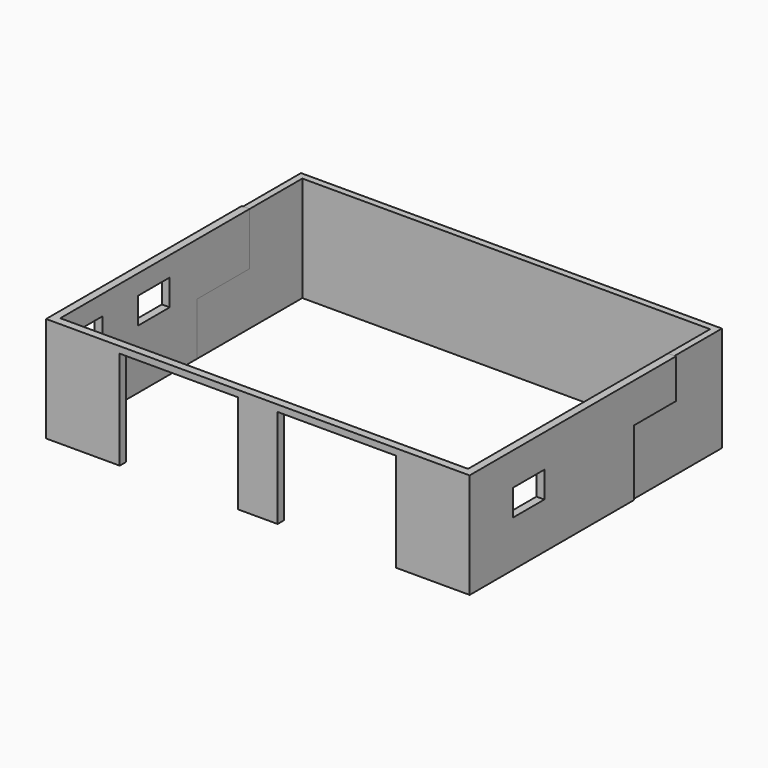
from build123d import *

# Parameters (mm, degrees)
F0_W           = 9753.6
F0_H           = 7315.2
F1_DEPTH       = 304.8
F2_W           = 914.4
F2_H           = 152.4
F3_DEPTH       = 152.4
F5_DEPTH       = 2438.4
F7_DEPTH       = 152.4
F9_DEPTH       = 152.4
F10_W          = 914.4
F10_H          = 609.6
F11_DEPTH      = 152.4
F11_DEPTH_BACK = 30.48
F13_DEPTH      = 152.4
F13_DEPTH_BACK = 30.48
F14_W          = 914.4
F14_H          = 609.6
F15_DEPTH      = 182.88
F16_W          = 9753.6
F16_H          = 7315.2
F17_DEPTH      = 457.5


with BuildPart() as f1:
    # F0 (on Top) → F1 (new body)
    with BuildSketch(Plane.XY):
        with Locations((4876.8, 3657.6)):
            Rectangle(F0_W, F0_H)
    extrude(amount=F1_DEPTH)

    # F2 (on face) → F3 (join)
    with BuildSketch(Plane.XY.offset(304.8)):
        with Locations((4876.8, 76.2)):
            Rectangle(F2_W, F2_H)
        Polygon((8077.2, 152.4), (8077.2, 0), (9753.6, 0), (9753.6, 7315.2), (0, 7315.2), (0, 1371.6), (152.4, 1371.6), (152.4, 7162.8), (9601.2, 7162.8), (9601.2, 152.4), align=None)
        Polygon((0, 0), (1676.4, 0), (1676.4, 152.4), (152.4, 152.4), (152.4, 457.2), (0, 457.2), align=None)
    extrude(amount=F3_DEPTH)

    # F4 (on face) → F5 (join)
    with BuildSketch(Plane.XY.offset(457.2)):
        Polygon((0, 7315.2), (0, 7162.8), (9601.2, 7162.8), (9753.6, 7162.8), (9753.6, 7315.2), align=None)
    extrude(amount=F5_DEPTH)

    # F6 (on face) → F7 (join)
    with BuildSketch(Plane.YZ.offset(9753.6)):
        Polygon((4724.4, 1981.2), (4724.4, 457.2), (7162.8, 457.2), (7162.8, 2895.6), (5943.6, 2895.6), (5943.6, 1981.2), align=None)
    extrude(amount=-F7_DEPTH)

    # F8 (on face) → F9 (join)
    with BuildSketch(Plane(origin=(0, 0, 0), x_dir=(0, -1, 0), z_dir=(-1, 0, 0))):
        Polygon((-7162.8, 457.2), (-4114.8, 457.2), (-4114.8, 1676.4), (-5638.8, 1676.4), (-5638.8, 2895.6), (-7162.8, 2895.6), align=None)
    extrude(amount=-F9_DEPTH)

    # F16 (on face) → F17 (cut)
    with BuildSketch(Plane(origin=(0, 0, 0), x_dir=(1, 0, 0), z_dir=(0, 0, -1))):
        with Locations((4876.8, -3657.6)):
            Rectangle(F16_W, F16_H)
    extrude(amount=-F17_DEPTH, mode=Mode.SUBTRACT)


with BuildPart() as f11:
    # F10 (on face) → F11 (new body, two sides)
    with BuildSketch(Plane.YZ.offset(9753.6)) as f11_sk:
        Polygon((5943.6, 1981.2), (5943.6, 2895.6), (0, 2895.6), (0, 457.2), (4724.4, 457.2), (4724.4, 1981.2), align=None)
        with Locations((1676.4, 1828.8)):
            Rectangle(F10_W, F10_H, mode=Mode.SUBTRACT)
    extrude(amount=-F11_DEPTH)
    extrude(f11_sk.sketch, amount=F11_DEPTH_BACK)

    # F12 (on face) → F13 (join, two sides)
    with BuildSketch(Plane.XZ) as f13_sk:
        Polygon((-30.48, 457.2), (0, 457.2), (1676.4, 457.2), (1676.4, 2743.2), (4419.6, 2743.2), (4419.6, 457.2), (5334, 457.2), (5334, 2743.2), (8077.2, 2743.2), (8077.2, 457.2), (9601.2, 457.2), (9753.6, 457.2), (9784.08, 457.2), (9784.08, 2895.6), (9601.2, 2895.6), (152.4, 2895.6), (-30.48, 2895.6), align=None)
    extrude(amount=-F13_DEPTH)
    extrude(f13_sk.sketch, amount=F13_DEPTH_BACK)

    # F14 (on face) → F15 (join)
    with BuildSketch(Plane(origin=(-30.48, 0, 0), x_dir=(0, -1, 0), z_dir=(-1, 0, 0))):
        Polygon((30.48, 2895.6), (-5638.8, 2895.6), (-5638.8, 1676.4), (-4114.8, 1676.4), (-4114.8, 457.2), (-1371.6, 457.2), (-1371.6, 2438.4), (-457.2, 2438.4), (-457.2, 457.2), (30.48, 457.2), align=None)
        with Locations((-2865.12, 2133.6)):
            Rectangle(F14_W, F14_H, mode=Mode.SUBTRACT)
    extrude(amount=-F15_DEPTH)


solid = Compound([f1.part, f11.part])
